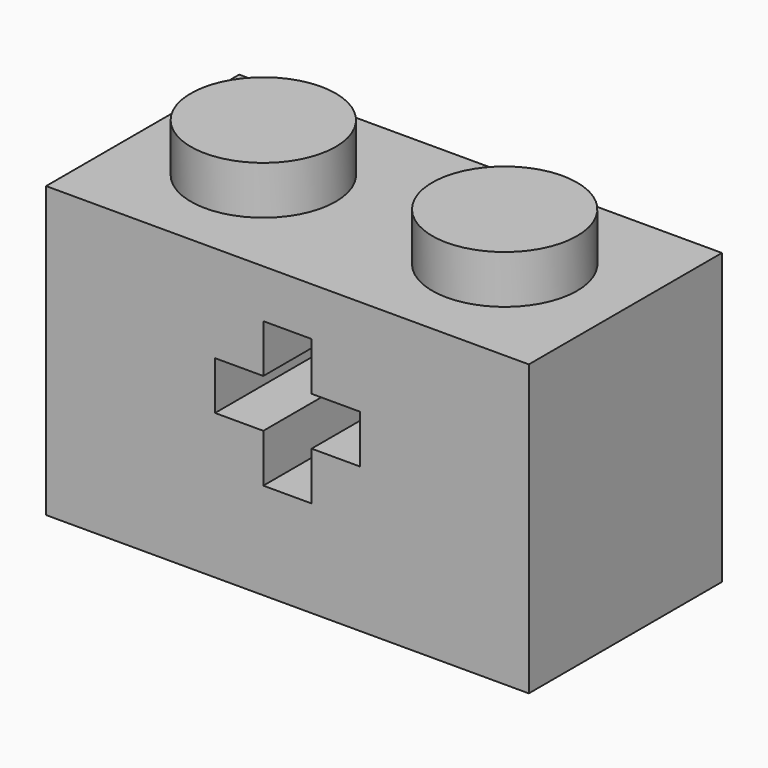
from build123d import *

# Parameters (mm, degrees)
F0_W        = 15.875
F0_H        = 9.525
F1_DEPTH    = 7.9375
F2_T        = 1.5875
F2_T3_DEPTH = 11.1125
F3_R        = 2.38125
F4_DEPTH    = 1.5875


# Not quite as in the source:
# - a shell that OpenCascade refuses in one call is made with other operations: the cavity is built on its own and cut out


with BuildPart() as f1:
    # F0 (on Front) → F1 (new body)
    with BuildSketch(Plane.XZ):
        Rectangle(F0_W, F0_H)
        Polygon((-0.79375, 1.5875), (-0.79375, 3.175), (0.79375, 3.175), (0.79375, 1.5875), (2.38125, 1.5875), (2.38125, 0), (0.79375, 0), (0.79375, -1.5875), (-0.79375, -1.5875), (-0.79375, 0), (-2.38125, 0), (-2.38125, 1.5875), align=None, mode=Mode.SUBTRACT)
    extrude(amount=F1_DEPTH)

    # F2: shell of thickness 1.5875, made by hand


with BuildPart() as f2_core1:
    # F2_t2: copy of F1
    add(f1.part)

    # the walls: a layer under each face that stays
    f2_faces = [f2_core1.faces().sort_by_distance(p)[0] for p in [
        (0, -3.96875, 4.7625),
        (-7.9375, -3.96875, 0),
        (7.9375, -3.96875, 0),
        (-0.79375, -3.96875, -0.79375),
        (-1.5875, -3.96875, 0),
        (-2.38125, -3.96875, 0.79375),
        (-1.5875, -3.96875, 1.5875),
        (-0.79375, -3.96875, 2.38125),
        (0, -3.96875, 3.175),
        (0.79375, -3.96875, 2.38125),
        (1.5875, -3.96875, 1.5875),
        (2.38125, -3.96875, 0.79375),
        (1.5875, -3.96875, 0),
        (0.79375, -3.96875, -0.79375),
        (0, -3.96875, -1.5875),
        (-5.2916666667, 0, -3.175),
        (-5.2916666667, -7.9375, -3.175),
    ]]
    thicken(f2_faces, amount=-F2_T, mode=Mode.SUBTRACT)

    # F2_s4 → F2_t3 (cut)
    with BuildSketch(Plane.XZ.offset(-1.5875)):
        Polygon((-0.777875, -1.571625), (-2.38125, -1.5875), (-2.38125, -3.175), (-0.79375, -3.175), align=None)
        Polygon((-2.365375, 0.015875), (-2.38125, -1.5875), (-3.96875, -1.5875), (-3.96875, 0), align=None)
        Polygon((-2.365375, 1.571625), (-3.96875, 1.5875), (-3.96875, 3.175), (-2.38125, 3.175), align=None)
        Polygon((-0.777875, 3.159125), (-2.38125, 3.175), (-2.38125, 4.7625), (-0.79375, 4.7625), align=None)
        Polygon((0.777875, 3.159125), (0.79375, 4.7625), (2.38125, 4.7625), (2.38125, 3.175), align=None)
        Polygon((2.365375, 1.571625), (2.38125, 3.175), (3.96875, 3.175), (3.96875, 1.5875), align=None)
        Polygon((2.365375, 0.015875), (3.96875, 0), (3.96875, -1.5875), (2.38125, -1.5875), align=None)
        Polygon((0.777875, -1.571625), (2.38125, -1.5875), (2.38125, -3.175), (0.79375, -3.175), align=None)
    extrude(amount=F2_T3_DEPTH, mode=Mode.SUBTRACT)


with BuildPart() as f1_1:
    add(f1.part)

    # what is left inside the walls is the cavity
    f2_cavity = [f2_core1.part.solids().sort_by_distance(p)[0] for p in [
        (0, -4.7625, -4.746625),
    ]]
    add(f2_cavity, mode=Mode.SUBTRACT)

    # F3 (on face) → F4 (join)
    with BuildSketch(Plane.XY.offset(4.7625)):
        with Locations((-3.96875, -3.96875)):
            Circle(F3_R)
        with Locations((3.96875, -3.96875)):
            Circle(F3_R)
    extrude(amount=F4_DEPTH)


solid = f1_1.part
